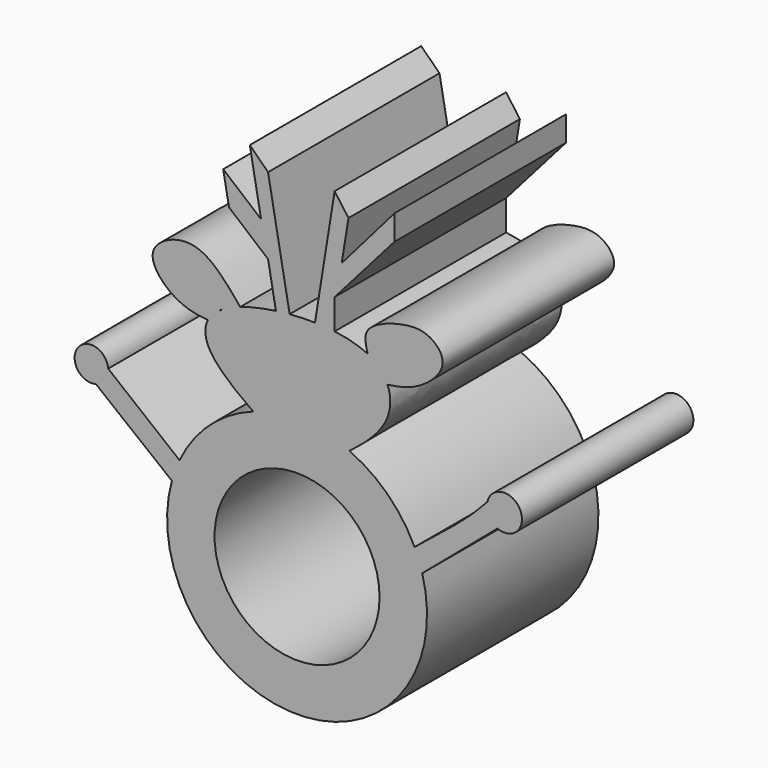
from build123d import *

# Parameters (mm, degrees)
F0_R     = 1.2343431581
F0_R_2   = 1.1676202912
F1_DEPTH = 25.4
F2_R     = 9.777673903
F3_DEPTH = 25.4010001


# Not quite as in the source:
# - a feature names something its author has since deleted; it is built from what else it names


with BuildPart() as f1:
    # F0 (on Front) → F1 (new body)
    with BuildSketch(Plane.XZ):
        with BuildLine():
            ThreePointArc((-1.9968199656, 7.5688475417), (0, 9.5656675073), (1.9968199656, 7.5688475417))
            add(Edge.make_bspline(
                [(3.2633473205, 8.4793044276), (2.841689417, 8.1773369558), (2.417681238, 7.8743128728), (1.9968199656, 7.5688475417)],
                knots=[0.9731401377, 0.9731401377, 0.9731401377, 0.9731401377, 1, 1, 1, 1], degree=3))
            add(Edge.make_bspline(
                [(5.291820418, 9.9603919059), (4.6380599048, 9.4654757695), (3.9538550257, 8.9738068766), (3.2633473205, 8.4793044276)],
                knots=[0.9291543812, 0.9291543812, 0.9291543812, 0.9291543812, 0.9731401377, 0.9731401377, 0.9731401377, 0.9731401377], degree=3))
            add(Edge.make_bspline(
                [(9.8224105557, 18.3403169376), (10.2657515128, 17.2671971534), (10.2057973933, 14.1054721398), (7.3643949931, 11.5293924505), (5.291820418, 9.9603919059)],
                knots=[0.7048700925, 0.7048700925, 0.7048700925, 0.7048700925, 0.7897091886, 0.9291543812, 0.9291543812, 0.9291543812, 0.9291543812], degree=3))
            add(Edge.make_bspline(
                [(9.0404523602, 19.5806321203), (9.3820768283, 19.1971335676), (9.6411804083, 18.7789898223), (9.8224105557, 18.3403169376)],
                knots=[0.6701893312, 0.6701893312, 0.6701893312, 0.6701893312, 0.7048700925, 0.7048700925, 0.7048700925, 0.7048700925], degree=3))
            add(Edge.make_bspline(
                [(9.0164794626, 19.6073366215), (9.0241449488, 19.5979806062), (9.0321349993, 19.5890743409), (9.0404523602, 19.5806321203)],
                knots=[0.9951430193, 0.9951430193, 0.9951430193, 0.9951430193, 1, 1, 1, 1], degree=3))
            add(Edge.make_bspline(
                [(7.4781377275, 20.7706270595), (8.1063529664, 20.4442707486), (8.6167334364, 20.0492172461), (9.0164794626, 19.6073366215)],
                knots=[0.6292527912, 0.6292527912, 0.6292527912, 0.6292527912, 0.6693826452, 0.6693826452, 0.6693826452, 0.6693826452], degree=3))
            add(Edge.make_bspline(
                [(3.5498395186, 21.8525875291), (5.0709035737, 21.6640168859), (6.4365000788, 21.3117553214), (7.4781377275, 20.7706270595)],
                knots=[0.562713866, 0.562713866, 0.562713866, 0.562713866, 0.6292527912, 0.6292527912, 0.6292527912, 0.6292527912], degree=3))
            add(Edge.make_bspline(
                [(1.2218726617, 22.0148384046), (2.0219718496, 21.9980775903), (2.8045671105, 21.9449810722), (3.5498395186, 21.8525875291)],
                knots=[0.5301119353, 0.5301119353, 0.5301119353, 0.5301119353, 0.562713866, 0.562713866, 0.562713866, 0.562713866], degree=3))
            add(Edge.make_bspline(
                [(-1.7825967517, 21.9164786942), (-0.7792787738, 22.0008787252), (0.2346221093, 22.0355197444), (1.2218726617, 22.0148384046)],
                knots=[0.4898840803, 0.4898840803, 0.4898840803, 0.4898840803, 0.5301119353, 0.5301119353, 0.5301119353, 0.5301119353], degree=3))
            add(Edge.make_bspline(
                [(-3.4071633919, 21.7351022024), (-2.8727981588, 21.8097333743), (-2.3292683633, 21.8704921755), (-1.7825967517, 21.9164786942)],
                knots=[0.4679653797, 0.4679653797, 0.4679653797, 0.4679653797, 0.4898840803, 0.4898840803, 0.4898840803, 0.4898840803], degree=3))
            add(Edge.make_bspline(
                [(-7.6403221771, 20.7706270595), (-6.3998054208, 21.1922572452), (-4.9412508039, 21.5208466068), (-3.4071633919, 21.7351022024)],
                knots=[0.4050398738, 0.4050398738, 0.4050398738, 0.4050398738, 0.4679653797, 0.4679653797, 0.4679653797, 0.4679653797], degree=3))
            add(Edge.make_bspline(
                [(-9.8129768452, 19.7946945944), (-9.2177162529, 20.158130564), (-8.4788283728, 20.4856333089), (-7.6403221771, 20.7706270595)],
                knots=[0.3625064487, 0.3625064487, 0.3625064487, 0.3625064487, 0.4050398738, 0.4050398738, 0.4050398738, 0.4050398738], degree=3))
            add(Edge.make_bspline(
                [(-9.8129768452, 19.7946945944), (-9.8626572034, 19.7193909877), (-9.9490587456, 19.6661416758), (-10.0647194767, 19.6331309022)],
                knots=[0, 0, 0, 0, 0.0391866891, 0.0391866891, 0.0391866891, 0.0391866891], degree=3))
            add(Edge.make_bspline(
                [(-11.4547769714, 18.1728920256), (-11.1799307011, 18.6961641136), (-10.722667508, 19.1889237515), (-10.0647194767, 19.6331309022)],
                knots=[0.3057347726, 0.3057347726, 0.3057347726, 0.3057347726, 0.3562922319, 0.3562922319, 0.3562922319, 0.3562922319], degree=3))
            add(Edge.make_bspline(
                [(-6.0977533046, 10.3582262113), (-8.6062536302, 12.1230052446), (-11.8222803026, 14.7501658532), (-11.892115865, 17.3402547999), (-11.4547769714, 18.1728920256)],
                knots=[0.0767336432, 0.0767336432, 0.0767336432, 0.0767336432, 0.2252870982, 0.3057347726, 0.3057347726, 0.3057347726, 0.3057347726], degree=3))
            add(Edge.make_bspline(
                [(-3.9700187942, 8.9003053831), (-4.698469629, 9.3913862847), (-5.4138065645, 9.877056305), (-6.0977533046, 10.3582262113)],
                knots=[0.0362302993, 0.0362302993, 0.0362302993, 0.0362302993, 0.0767336432, 0.0767336432, 0.0767336432, 0.0767336432], degree=3))
            add(Edge.make_bspline(
                [(-1.9968199656, 7.5688475417), (-2.6563252964, 8.0174308154), (-3.3184184759, 8.4610328111), (-3.9700187942, 8.9003053831)],
                knots=[0, 0, 0, 0, 0.0362302993, 0.0362302993, 0.0362302993, 0.0362302993], degree=3))
        make_face()
        with Locations((-2.5474067745, 12.413466867)):
            Circle(F0_R, mode=Mode.SUBTRACT)
        with Locations((1.6244133145, 12.2344455942)):
            Circle(F0_R_2, mode=Mode.SUBTRACT)
        with BuildLine():
            ThreePointArc((-1.9968199656, 7.5688475417), (0, 5.5720275761), (1.9968199656, 7.5688475417))
            ThreePointArc((1.9968199656, 7.5688475417), (0, 9.5656675073), (-1.9968199656, 7.5688475417))
        make_face()
        with BuildLine():
            add(Edge.make_bspline(
                [(-11.4547769714, 18.1728920256), (-13.2618411574, 18.2583922451), (-16.1819405075, 19.1885835024), (-19.4228561636, 23.6007697874), (-12.8090262125, 26.9600135992), (-9.4729623186, 23.020656954), (-7.6403221771, 20.7706270595)],
                knots=[0, 0, 0, 0, 0.2429778163, 0.4587446686, 0.6993896075, 1, 1, 1, 1], degree=3))
            add(Edge.make_bspline(
                [(-11.4547769714, 18.1728920256), (-11.1799307011, 18.6961641136), (-10.722667508, 19.1889237515), (-10.0647194767, 19.6331309022)],
                knots=[0.3057347726, 0.3057347726, 0.3057347726, 0.3057347726, 0.3562922319, 0.3562922319, 0.3562922319, 0.3562922319], degree=3))
            add(Edge.make_bspline(
                [(-10.0647194767, 19.6331309022), (-10.7420183544, 19.4398227702), (-14.127166026, 20.448341035), (-16.206710897, 23.9906258668), (-11.9787863154, 23.137781592), (-9.4800821705, 20.299283743), (-9.8129768452, 19.7946945944)],
                knots=[0.0391866891, 0.0391866891, 0.0391866891, 0.0391866891, 0.2686604293, 0.5013914501, 0.7374205704, 1, 1, 1, 1], degree=3))
            add(Edge.make_bspline(
                [(-9.8129768452, 19.7946945944), (-9.2177162529, 20.158130564), (-8.4788283728, 20.4856333089), (-7.6403221771, 20.7706270595)],
                knots=[0.3625064487, 0.3625064487, 0.3625064487, 0.3625064487, 0.4050398738, 0.4050398738, 0.4050398738, 0.4050398738], degree=3))
        make_face()
        with BuildLine():
            Line((-4.3387768686, 26.8339979934), (-3.4071633919, 21.7351022024))
            add(Edge.make_bspline(
                [(-3.4071633919, 21.7351022024), (-2.8727981588, 21.8097333743), (-2.3292683633, 21.8704921755), (-1.7825967517, 21.9164786942)],
                knots=[0.4679653797, 0.4679653797, 0.4679653797, 0.4679653797, 0.4898840803, 0.4898840803, 0.4898840803, 0.4898840803], degree=3))
            Line((-1.7825967517, 21.9164786942), (-4.3387768686, 35.9069332823))
            Line((-4.3387768686, 35.9069332823), (-6.5032765269, 38.0355417728))
            Line((-6.5032765269, 38.0355417728), (-5.1694188174, 30.7350876349))
            Line((-5.1694188174, 30.7350876349), (-9.6563799307, 34.4880223274))
            Line((-9.6563799307, 34.4880223274), (-8.9706854823, 30.7350876349))
            Line((-8.9706854823, 30.7350876349), (-4.3387768686, 26.8339979934))
        make_face()
        with BuildLine():
            add(Edge.make_bspline(
                [(-10.0647194767, 19.6331309022), (-10.7420183544, 19.4398227702), (-14.127166026, 20.448341035), (-16.206710897, 23.9906258668), (-11.9787863154, 23.137781592), (-9.4800821705, 20.299283743), (-9.8129768452, 19.7946945944)],
                knots=[0.0391866891, 0.0391866891, 0.0391866891, 0.0391866891, 0.2686604293, 0.5013914501, 0.7374205704, 1, 1, 1, 1], degree=3))
            add(Edge.make_bspline(
                [(-10.0647194767, 19.6331309022), (-9.9838484879, 19.687730156), (-9.899945585, 19.7415958866), (-9.8129768452, 19.7946945944)],
                knots=[0.3562922319, 0.3562922319, 0.3562922319, 0.3562922319, 0.3625064487, 0.3625064487, 0.3625064487, 0.3625064487], degree=3))
        make_face()
        with BuildLine():
            add(Edge.make_bspline(
                [(1.2218726617, 22.0148384046), (2.0219718496, 21.9980775903), (2.8045671105, 21.9449810722), (3.5498395186, 21.8525875291)],
                knots=[0.5301119353, 0.5301119353, 0.5301119353, 0.5301119353, 0.562713866, 0.562713866, 0.562713866, 0.562713866], degree=3))
            Line((3.5498395186, 21.8525875291), (3.5498395186, 25.4404416609))
            Line((3.5498395186, 25.4404416609), (10.6439810566, 33.5208887535))
            Line((10.6439810566, 33.5208887535), (10.6439810566, 36.4897335443))
            Line((10.6439810566, 36.4897335443), (4.3906857101, 29.2522859745))
            Line((4.3906857101, 29.2522859745), (5.1904305148, 34.224960801))
            Line((5.1904305148, 34.224960801), (3.5498395186, 36.4897335443))
            Line((3.5498395186, 36.4897335443), (1.2218726617, 22.0148384046))
        make_face()
        with BuildLine():
            add(Edge.make_bspline(
                [(9.0404523602, 19.5806321203), (9.3820768283, 19.1971335676), (9.6411804083, 18.7789898223), (9.8224105557, 18.3403169376)],
                knots=[0.6701893312, 0.6701893312, 0.6701893312, 0.6701893312, 0.7048700925, 0.7048700925, 0.7048700925, 0.7048700925], degree=3))
            add(Edge.make_bspline(
                [(9.8224105557, 18.3403169376), (11.2153140722, 18.5109801218), (13.7892848388, 19.1004981723), (17.2606461127, 22.5302099032), (15.0050826028, 25.2706081918), (11.9173641085, 25.5467387461), (6.6576478669, 23.7334481834), (7.2324744651, 21.6701568434), (7.4781377275, 20.7706270595)],
                knots=[0, 0, 0, 0, 0.1822400506, 0.3612657036, 0.5045524169, 0.663892651, 0.8591676122, 1, 1, 1, 1], degree=3))
            add(Edge.make_bspline(
                [(7.4781377275, 20.7706270595), (8.1063529664, 20.4442707486), (8.6167334364, 20.0492172461), (9.0164794626, 19.6073366215)],
                knots=[0.6292527912, 0.6292527912, 0.6292527912, 0.6292527912, 0.6693826452, 0.6693826452, 0.6693826452, 0.6693826452], degree=3))
            add(Edge.make_bspline(
                [(9.0404523602, 19.5806321203), (9.4784020758, 19.1361079274), (12.0293402458, 20.7326500765), (13.9949567764, 23.4997662714), (9.668194415, 23.7104945441), (8.5939298141, 20.1230744252), (9.0164794626, 19.6073366215)],
                knots=[0, 0, 0, 0, 0.255743784, 0.4848908681, 0.7274084652, 0.9951430193, 0.9951430193, 0.9951430193, 0.9951430193], degree=3))
        make_face()
        with BuildLine():
            add(Edge.make_bspline(
                [(9.0164794626, 19.6073366215), (9.0245151148, 19.598453984), (9.0325060612, 19.5895524244), (9.0404523602, 19.5806321203)],
                knots=[0.6693826452, 0.6693826452, 0.6693826452, 0.6693826452, 0.6701893312, 0.6701893312, 0.6701893312, 0.6701893312], degree=3))
            add(Edge.make_bspline(
                [(9.0404523602, 19.5806321203), (9.4784020758, 19.1361079274), (12.0293402458, 20.7326500765), (13.9949567764, 23.4997662714), (9.668194415, 23.7104945441), (8.5939298141, 20.1230744252), (9.0164794626, 19.6073366215)],
                knots=[0, 0, 0, 0, 0.255743784, 0.4848908681, 0.7274084652, 0.9951430193, 0.9951430193, 0.9951430193, 0.9951430193], degree=3))
        make_face()
        with Locations((1.6244133145, 12.2344455942)):
            Circle(F0_R_2)
        with Locations((-2.5474067745, 12.413466867)):
            Circle(F0_R)
        with BuildLine():
            add(Edge.make_bspline(
                [(3.2633473205, 8.4793044276), (2.841689417, 8.1773369558), (2.417681238, 7.8743128728), (1.9968199656, 7.5688475417)],
                knots=[0.9731401377, 0.9731401377, 0.9731401377, 0.9731401377, 1, 1, 1, 1], degree=3))
            ThreePointArc((1.9968199656, 7.5688475417), (0, 5.5720275761), (-1.9968199656, 7.5688475417))
            add(Edge.make_bspline(
                [(-1.9968199656, 7.5688475417), (-2.6563252964, 8.0174308154), (-3.3184184759, 8.4610328111), (-3.9700187942, 8.9003053831)],
                knots=[0, 0, 0, 0, 0.0362302993, 0.0362302993, 0.0362302993, 0.0362302993], degree=3))
            add(Edge.make_bspline(
                [(-3.9700187942, 8.9003053831), (-6.9902118362, 5.8201430862), (-12.8862109887, 0.4369124192), (-11.7946728285, -6.7063142641), (-9.2590422156, -17.5990966335), (-6.1766836432, -4.8008390766), (-1.1883774497, -21.4983309099), (-1.4966768799, -5.6799294478), (8.3885389188, -20.2079907911), (4.1770733312, -2.7890633953), (11.961574095, -14.0816381699), (8.986776897, -0.572525648), (13.2777598832, -8.0107441312), (11.4445848325, 4.674510475), (6.1620931725, 7.1594239129), (3.2633473205, 8.4793044276)],
                knots=[0, 0, 0, 0, 0.1016288045, 0.1850105958, 0.2605805278, 0.3277901899, 0.4097509261, 0.481040342, 0.5604810392, 0.6410163658, 0.7044948285, 0.7793548179, 0.825264206, 0.9078715102, 1, 1, 1, 1], degree=3))
        make_face()
        with BuildLine():
            add(Edge.make_bspline(
                [(5.291820418, 9.9603919059), (4.6380599048, 9.4654757695), (3.9538550257, 8.9738068766), (3.2633473205, 8.4793044276)],
                knots=[0.9291543812, 0.9291543812, 0.9291543812, 0.9291543812, 0.9731401377, 0.9731401377, 0.9731401377, 0.9731401377], degree=3))
            add(Edge.make_bspline(
                [(-3.9700187942, 8.9003053831), (-6.9902118362, 5.8201430862), (-12.8862109887, 0.4369124192), (-11.7946728285, -6.7063142641), (-9.2590422156, -17.5990966335), (-6.1766836432, -4.8008390766), (-1.1883774497, -21.4983309099), (-1.4966768799, -5.6799294478), (8.3885389188, -20.2079907911), (4.1770733312, -2.7890633953), (11.961574095, -14.0816381699), (8.986776897, -0.572525648), (13.2777598832, -8.0107441312), (11.4445848325, 4.674510475), (6.1620931725, 7.1594239129), (3.2633473205, 8.4793044276)],
                knots=[0, 0, 0, 0, 0.1016288045, 0.1850105958, 0.2605805278, 0.3277901899, 0.4097509261, 0.481040342, 0.5604810392, 0.6410163658, 0.7044948285, 0.7793548179, 0.825264206, 0.9078715102, 1, 1, 1, 1], degree=3))
            add(Edge.make_bspline(
                [(-3.9700187942, 8.9003053831), (-4.698469629, 9.3913862847), (-5.4138065645, 9.877056305), (-6.0977533046, 10.3582262113)],
                knots=[0.0362302993, 0.0362302993, 0.0362302993, 0.0362302993, 0.0767336432, 0.0767336432, 0.0767336432, 0.0767336432], degree=3))
            ThreePointArc((-6.0977533046, 10.3582262113), (-11.2522703526, 7.2663125794), (-14.8312818353, 2.4372699504))
            Line((-14.8312818353, 2.4372699504), (-23.2887535927, 9.2411445911))
            ThreePointArc((-23.2887535927, 9.2411445911), (-26.9055674019, 10.2310859611), (-24.7547028528, 7.1594239129))
            Line((-24.7547028528, 7.1594239129), (-15.7401796902, 0))
            ThreePointArc((-15.7401796902, 0), (-0.9026138185, -19.5507430015), (13.9349520533, 0))
            Line((13.9349520533, 0), (22.8549973194, 7.5688475417))
            ThreePointArc((22.8549973194, 7.5688475417), (25.5333188907, 10.4197188603), (21.6487478123, 9.9603919059))
            add(Edge.make_bspline(
                [(13.0260541983, 2.4372699504), (15.3164169129, 4.298441963), (19.2653346729, 7.3244846795), (20.9658887146, 9.2411445911), (21.6487478123, 9.9603919059)],
                knots=[0, 0, 0, 0, 0.6081778742, 1, 1, 1, 1], degree=3))
            ThreePointArc((13.0260541983, 2.4372699504), (9.8390877256, 6.8980675437), (5.291820418, 9.9603919059))
        make_face()
    extrude(amount=F1_DEPTH)

    # F2 (on face) → F3 (cut, through all)
    with BuildSketch(Plane.XZ.offset(25.4)):
        with Locations((-0.9026138185, -4.14506474)):
            Circle(F2_R)
    extrude(amount=-F3_DEPTH, mode=Mode.SUBTRACT)


solid = f1.part
